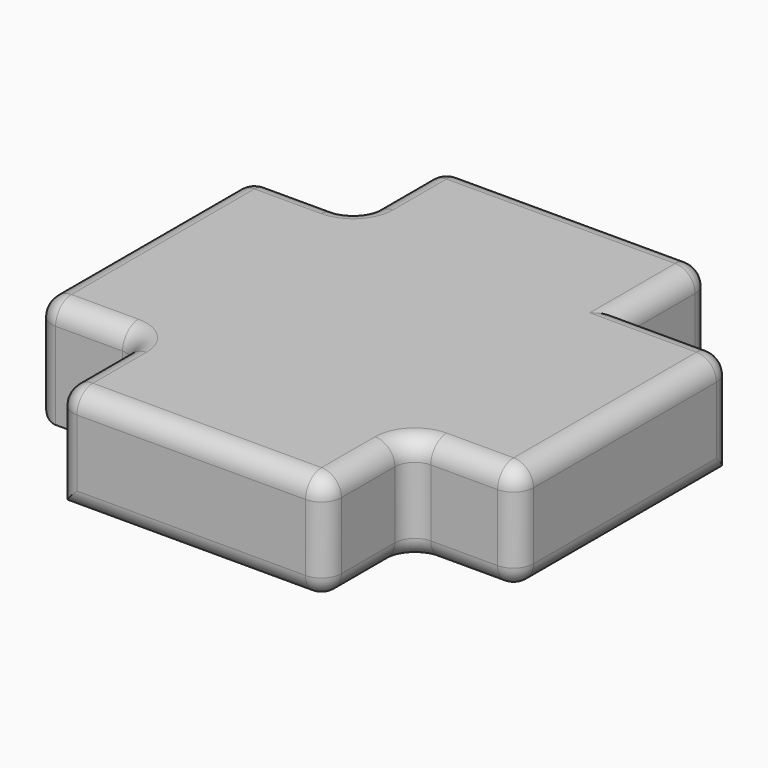
from build123d import *

# Parameters (mm, degrees)
F1_DEPTH = 26.8
F2_R     = 5


with BuildPart() as f1:
    # F0 (on Top) → F1 (new body)
    with BuildSketch(Plane.XY):
        Polygon((55.8652869582, 39.3723181486), (-11.5347130418, 39.3723181486), (-11.5347130418, 12.5723181486), (-38.3347130418, 12.5723181486), (-38.3347130418, -54.8276818514), (-11.5347130418, -54.8276818514), (-11.5347130418, -81.6276818514), (55.8652869582, -81.6276818514), (55.8652869582, -54.8276818514), (82.6652869582, -54.8276818514), (82.6652869582, 12.5723181486), (55.8652869582, 12.5723181486), align=None)
    extrude(amount=F1_DEPTH)

    # F2
    f2_edges = [f1.edges().sort_by_distance(p)[0] for p in [
        (-11.534713, -68.227682, 26.8),
        (22.165287, -81.627682, 26.8),
        (55.865287, -68.227682, 26.8),
        (69.265287, -54.827682, 26.8),
        (82.665287, -21.127682, 26.8),
        (69.265287, 12.572318, 26.8),
        (55.865287, 25.972318, 26.8),
        (22.165287, 39.372318, 26.8),
        (-11.534713, 25.972318, 26.8),
        (-24.934713, 12.572318, 26.8),
        (-38.334713, -21.127682, 26.8),
        (-24.934713, -54.827682, 26.8),
        (55.865287, -81.627682, 13.4),
        (55.865287, -54.827682, 13.4),
        (82.665287, -54.827682, 13.4),
        (82.665287, 12.572318, 13.4),
        (82.665287, -21.127682, 0),
        (-11.534713, -81.627682, 13.4),
        (22.165287, -81.627682, 0),
        (-11.534713, -54.827682, 13.4),
        (69.265287, -54.827682, 0),
        (-38.334713, 12.572318, 13.4),
        (-38.334713, -54.827682, 13.4),
        (-38.334713, -21.127682, 0),
        (-11.534713, 39.372318, 13.4),
        (-11.534713, 12.572318, 13.4),
        (-11.534713, 25.972318, 0),
        (55.865287, 39.372318, 13.4),
        (22.165287, 39.372318, 0),
        (55.865287, -68.227682, 0),
        (-24.934713, 12.572318, 0),
    ]]
    fillet(f2_edges, radius=F2_R)


solid = f1.part
